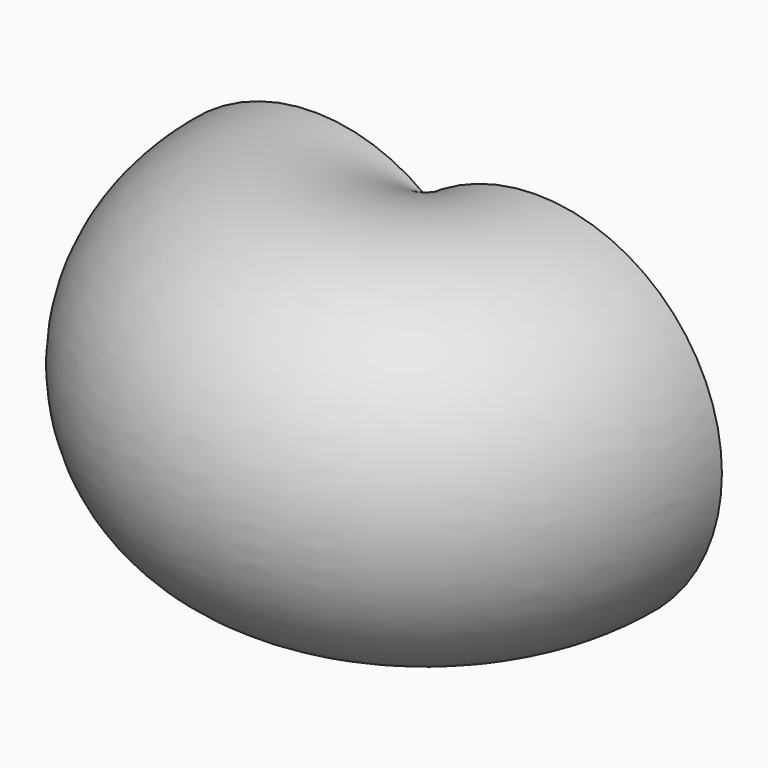
from build123d import *

# Parameters (mm, degrees)
F1_ANGLE = 180.2945364263


# Not quite as in the source:
# - the program builds the solid bodies; features that only make, move or delete a surface that nothing else refers to are left out


with BuildPart() as f1:
    # F0 (on Front) → F1 (revolve)
    with BuildSketch(Plane.XZ):
        with BuildLine():
            Line((0, 40), (0, 0))
            ThreePointArc((0, 0), (40, 20), (0, 40))
        make_face()
    revolve(axis=Axis((0, 0, 20), (0, 0, -1)), revolution_arc=F1_ANGLE)


solid = f1.part
